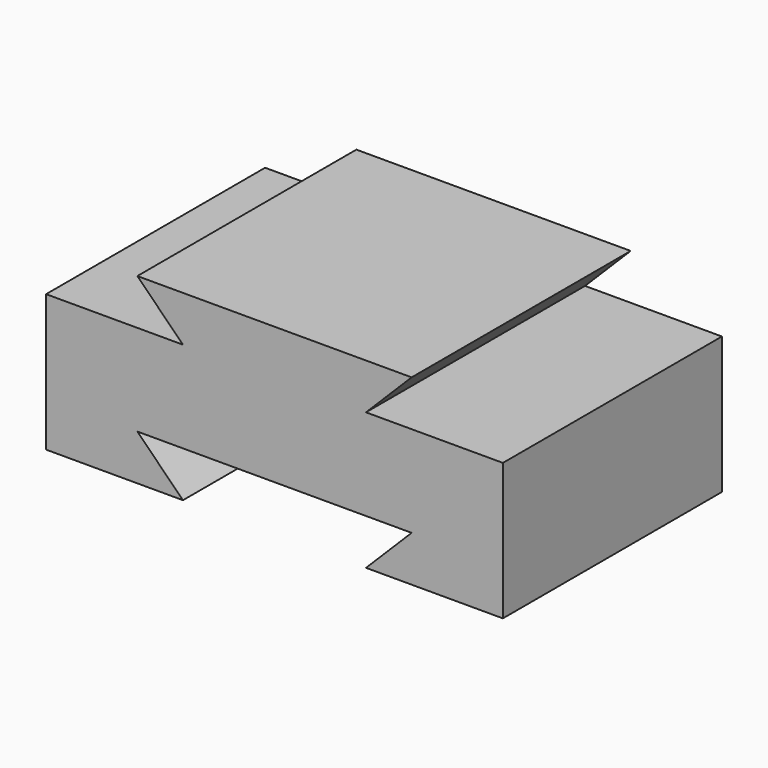
from build123d import *

# Parameters (mm, degrees)
F0_W     = 38.1
F0_H     = 76.2
F1_DEPTH = 12.7
F2_SIZE  = 12.69999
F3_W     = 76.2
F3_H     = 76.2
F4_DEPTH = 25.4
F5_W     = 50.8
F5_H     = 76.2
F6_DEPTH = 12.7
F8_DEPTH = 76.201


# Not quite as in the source:
# - a fillet or chamfer is up to 0.001 mm smaller than in the source, because OpenCascade refuses the exact size


with BuildPart() as f1:
    # F0 (on Top) → F1 (new body)
    with BuildSketch(Plane.XY):
        with Locations((-44.5209794172, 0.8258419111)):
            Rectangle(F0_W, F0_H)
    extrude(amount=F1_DEPTH)

    # F2 (size 12.7 in the source; OpenCascade refuses exactly that, so slightly less here)
    f2_edges = [f1.edges().sort_by_distance(p)[0] for p in [
        (-25.470979, 0.825842, 12.7),
    ]]
    chamfer(f2_edges, length=F2_SIZE)

    # F3 (on face) → F4 (join)
    with BuildSketch(Plane.XY.offset(12.7)):
        with Locations((-25.4709794172, 0.8258419111)):
            Rectangle(F3_W, F3_H)
    extrude(amount=F4_DEPTH)

    # F5 (on face) → F6 (join)
    with BuildSketch(Plane.XY.offset(38.1)):
        with Locations((-12.7709794172, 0.8258419111)):
            Rectangle(F5_W, F5_H)
    extrude(amount=F6_DEPTH)

    # F7 (on face) → F8 (cut, through all)
    with BuildSketch(Plane.XZ.offset(37.2741580889)):
        Polygon((-38.1709794172, 50.8), (-38.1709794172, 38.1), (-25.4709794172, 38.1), align=None)
    extrude(amount=-F8_DEPTH, mode=Mode.SUBTRACT)

    # F9: F1 across plane


with BuildPart() as f1_1:
    add(f1.part)
    add(f1.part.mirror(Plane.YZ))


solid = f1_1.part
